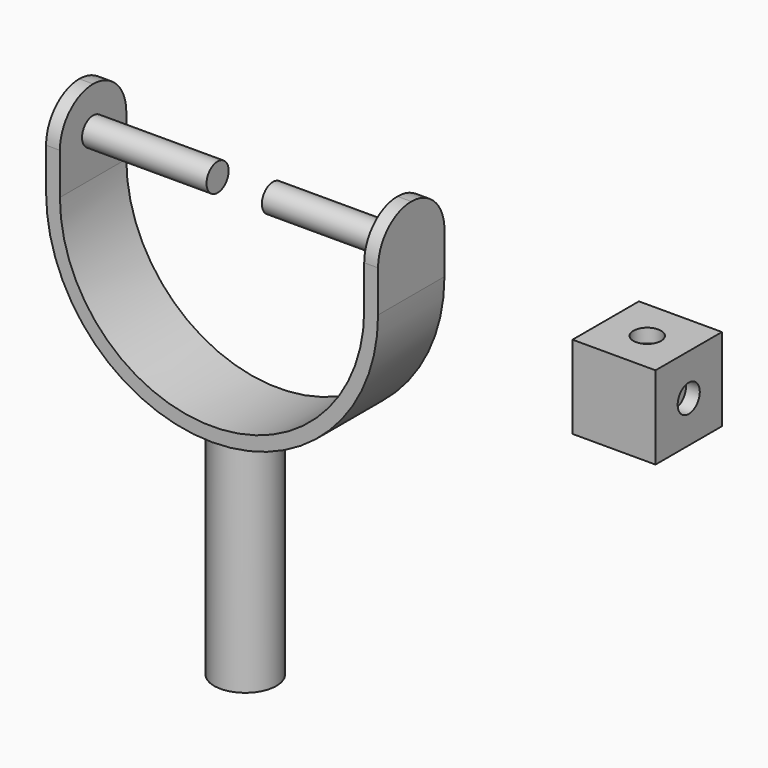
from build123d import *

# Parameters (mm, degrees)
F1_DEPTH  = 38.1
F2_DEPTH  = 38.1
F3_R      = 19.04999
F4_R      = 6.35
F5_DEPTH  = 69.85
F6_R      = 6.35
F7_DEPTH  = 12.7
F10_DEPTH = 115.6514373633
F11_DEPTH = 12.7
F12_W     = 38.1
F12_H     = 38.1
F13_DEPTH = 38.1
F14_R     = 6.35
F15_DEPTH = 6.35
F16_R     = 6.35
F17_DEPTH = 6.35
F18_R     = 6.35
F19_DEPTH = 6.35
F20_R     = 6.35
F21_DEPTH = 6.35


# Not quite as in the source:
# - a fillet or chamfer is up to 0.001 mm smaller than in the source, because OpenCascade refuses the exact size


with BuildPart() as f1:
    # F0 (on Front) → F1 (new body)
    with BuildSketch(Plane.XZ):
        with BuildLine():
            Line((-69.85, 0), (-76.2, 0))
            ThreePointArc((-76.2, 0), (0, -76.2), (76.2, 0))
            Line((76.2, 0), (69.85, 0))
            ThreePointArc((69.85, 0), (0, -69.85), (-69.85, 0))
        make_face()
    extrude(amount=F1_DEPTH)

    # F2 (add): faces of the model
    f2_faces = [f1.faces().sort_by_distance(p)[0] for p in [
        (73.025, -19.05, 0),
        (-73.025, -19.05, 0),
    ]]
    extrude(f2_faces, amount=F2_DEPTH)

    # F3 (radius 19.05 in the source; OpenCascade refuses exactly that, so slightly less here)
    f3_edges = [f1.edges().sort_by_distance(p)[0] for p in [
        (73.025, -38.1, 38.1),
        (73.025, 0, 38.1),
        (-73.025, 0, 38.1),
        (-73.025, -38.1, 38.1),
    ]]
    fillet(f3_edges, radius=F3_R)

    # F4 (on Right) → F5 (join, symmetric)
    with BuildSketch(Plane.YZ):
        with Locations((-19.05, 19.05)):
            Circle(F4_R)
    extrude(amount=F5_DEPTH, both=True)

    # F6 (on Right) → F7 (cut, symmetric)
    with BuildSketch(Plane.YZ):
        with Locations((-19.05, 19.05)):
            Circle(F6_R)
    extrude(amount=F7_DEPTH, both=True, mode=Mode.SUBTRACT)

    # F9 (on offset) → F10 (join, through all)
    with BuildSketch(Plane.XY.offset(-190.5)):
        with BuildLine():
            ThreePointArc((14.2875, -19.05), (10.1027881362, -8.9472118638), (0, -4.7625))
            ThreePointArc((0, -4.7625), (-10.1027881362, -29.1527881362), (14.2875, -19.05))
        make_face()
    extrude(amount=F10_DEPTH)

    # F11 (cut): a face of the model
    f11_faces = [f1.faces().sort_by_distance(p)[0] for p in [
        (0, -19.05, -190.5),
    ]]
    extrude(f11_faces, amount=-F11_DEPTH, mode=Mode.SUBTRACT)


with BuildPart() as f13:
    # F12 (on Front) → F13 (new body)
    with BuildSketch(Plane.XZ):
        with Locations((184.5231820917, 0)):
            Rectangle(F12_W, F12_H)
    extrude(amount=F13_DEPTH)

    # F14 (on face) → F15 (cut)
    with BuildSketch(Plane.YZ.offset(203.5731820917)):
        with Locations((-19.05, 0)):
            Circle(F14_R)
    extrude(amount=-F15_DEPTH, mode=Mode.SUBTRACT)

    # F16 (on face) → F17 (cut)
    with BuildSketch(Plane(origin=(165.4731820917, 0, 0), x_dir=(0, -1, 0), z_dir=(-1, 0, 0))):
        with Locations((19.05, 0)):
            Circle(F16_R)
    extrude(amount=-F17_DEPTH, mode=Mode.SUBTRACT)

    # F18 (on face) → F19 (cut)
    with BuildSketch(Plane.XY.offset(19.05)):
        with Locations((184.5231820917, -19.05)):
            Circle(F18_R)
    extrude(amount=-F19_DEPTH, mode=Mode.SUBTRACT)

    # F20 (on face) → F21 (cut)
    with BuildSketch(Plane(origin=(0, 0, -19.05), x_dir=(1, 0, 0), z_dir=(0, 0, -1))):
        with Locations((184.5231820917, 19.05)):
            Circle(F20_R)
    extrude(amount=-F21_DEPTH, mode=Mode.SUBTRACT)


solid = Compound([f1.part, f13.part])
